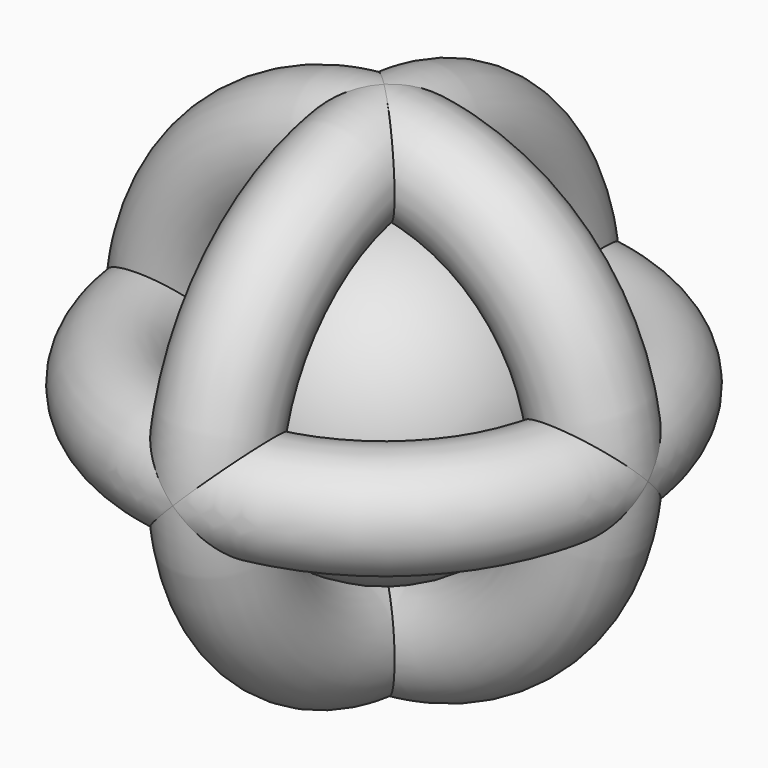
from build123d import *

# Parameters (mm, degrees)
F0_R = 12.7
F5_R = 12.7


with BuildPart() as f3:
    # F3: sweep along a path in F1
    with BuildLine(Plane.YZ) as f3_path:
        CenterArc((0, 0), 50.8, 0, 360)
    # F0 (on Front) → F3 (sweep)
    with BuildSketch(Plane.XZ):
        with Locations((0, 50.8)):
            Circle(F0_R)
    sweep(path=f3_path.line)

    # F4: sweep along a path in F2
    with BuildLine(Plane.XY) as f4_path:
        CenterArc((0, 0), 50.8, 0, 360)
    # F0 (on Front) → F4 (sweep)
    with BuildSketch(Plane.XZ):
        with Locations((50.8, 0)):
            Circle(F0_R)
    sweep(path=f4_path.line)

    # F7: sweep along a path in F6
    with BuildLine(Plane.XZ) as f7_path:
        CenterArc((0, 0), 50.8, 0, 360)
    # F5 (on Right) → F7 (sweep)
    with BuildSketch(Plane.YZ):
        with Locations((0, -50.8)):
            Circle(F5_R)
    sweep(path=f7_path.line)


with BuildPart() as f9:
    # F8 (on Top) → F9 (revolve)
    with BuildSketch(Plane.XY):
        with BuildLine():
            Line((0, 38.1), (0, -38.1))
            ThreePointArc((0, -38.1), (38.1, 0), (0, 38.1))
        make_face()
    revolve(axis=Axis((0, 0, 0), (0, -1, 0)))


solid = Compound([f3.part, f9.part])
